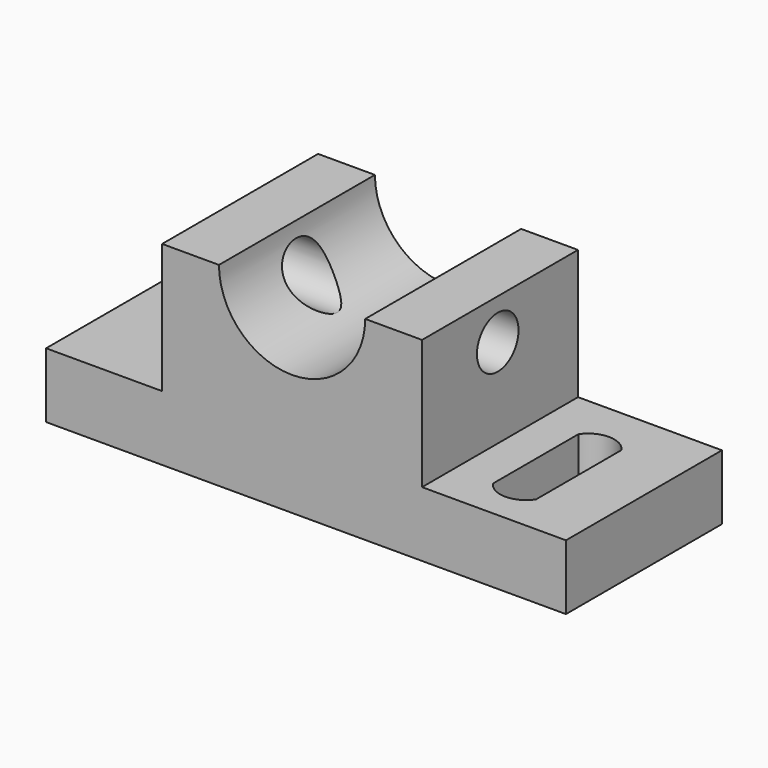
from build123d import *

# Parameters (mm, degrees)
F0_W     = 80
F0_H     = 39.8877346888
F1_DEPTH = 60
F3_DEPTH = 60.001
F5_DEPTH = 20.001
F6_R     = 8
F7_DEPTH = 115.7102386484


# Not quite as in the source:
# - a feature names something its author has since deleted; it is built from what else it names


with BuildPart() as f1:
    # F0 (on Front) → F1 (new body)
    with BuildSketch(Plane.XZ):
        with Locations((0, -35.378112942)):
            Rectangle(F0_W, F0_H)
        Polygon((-75.7092386484, -55.3219802864), (-75.7092386484, -75.3219802864), (84.2907613516, -75.3219802864), (84.2907613516, -55.3219802864), (40, -55.3219802864), (-40, -55.3219802864), align=None)
    extrude(amount=F1_DEPTH)

    # F2 (on face) → F3 (cut, through all)
    with BuildSketch(Plane.XZ.offset(60)):
        with BuildLine():
            Line((-22.5, -15.4342455976), (22.5, -15.4342455976))
            ThreePointArc((22.5, -15.4342455976), (0, 7.0657544024), (-22.5, -15.4342455976))
        make_face()
        with BuildLine():
            ThreePointArc((-22.5, -15.4342455976), (0, -37.9342455976), (22.5, -15.4342455976))
            Line((22.5, -15.4342455976), (-22.5, -15.4342455976))
        make_face()
    extrude(amount=-F3_DEPTH, mode=Mode.SUBTRACT)

    # F4 (on face) → F5 (cut, through all)
    with BuildSketch(Plane.XY.offset(-55.3219802864)):
        with BuildLine():
            Line((65.3745657473, -47.8825420141), (65.3745657473, -15.0121450424))
            ThreePointArc((65.3745657473, -15.0121450424), (58.7502594426, -11.4975174886), (52.1259531379, -15.0121450424))
            Line((52.1259531379, -15.0121450424), (52.1259531379, -47.8825420141))
            ThreePointArc((52.1259531379, -47.8825420141), (58.7502594426, -51.3971695679), (65.3745657473, -47.8825420141))
        make_face()
    extrude(amount=-F5_DEPTH, mode=Mode.SUBTRACT)

    # F6 (on face) → F7 (cut, through all)
    with BuildSketch(Plane.YZ.offset(40)):
        with Locations((-30.8821926572, -27.8876808805)):
            Circle(F6_R)
    extrude(amount=-F7_DEPTH, mode=Mode.SUBTRACT)


solid = f1.part
